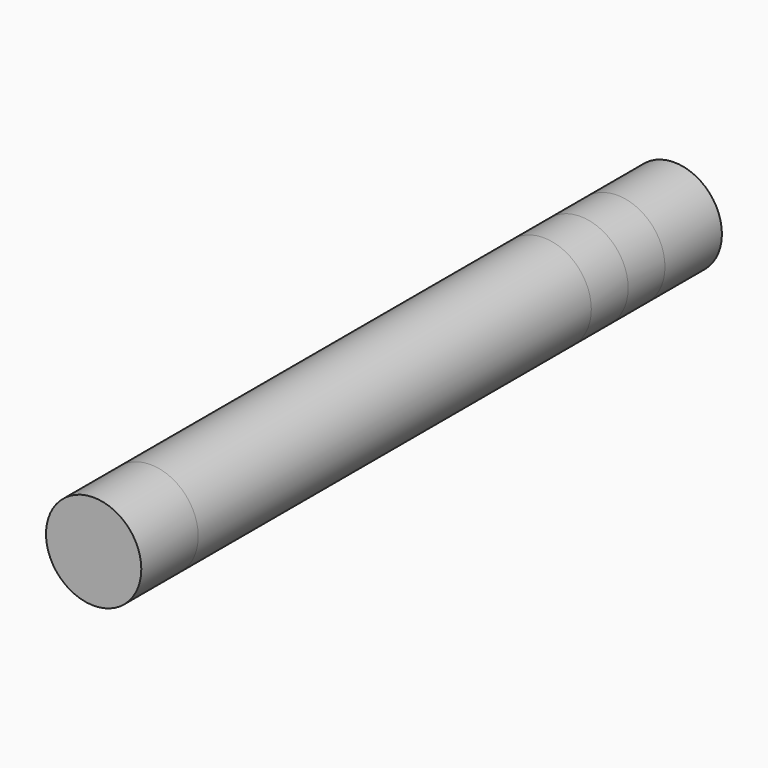
from build123d import *

# Parameters (mm, degrees)
F0_R          = 26.2972038965
F0_R_2        = 21.7596703079
F1_DEPTH      = 25.4
F2_DEPTH      = 25.4
F3_DEPTH      = 50.801
F3_DEPTH_BACK = 310.4061427


# Not quite as in the source:
# - an extrude ends at something that could not be found from the text; its depth is read off the source's solid
# - a feature of the source that left no trace in its solid (it failed there, or was rolled back) is left out
# - a pattern or mirror of a feature is missing from the dataset's text; its kind, count and spacing are read off the source's solid


with BuildPart() as f1:
    # F0 (on Front) → F1 (new body)
    with BuildSketch(Plane.XZ):
        with Locations((35.550635308, 42.1431325376)):
            Circle(F0_R)
        with Locations((35.550635308, 42.1431325376)):
            Circle(F0_R_2, mode=Mode.SUBTRACT)
        with Locations((35.550635308, 42.1431325376)):
            Circle(F0_R_2)
    extrude(amount=-F1_DEPTH)

    # F2 (add): a face of the model
    f2_faces = [f1.faces().sort_by_distance(p)[0] for p in [
        (35.550635308, 0, 42.1431325376),
    ]]
    extrude(f2_faces, amount=F2_DEPTH)

    # F3 (add, two sides): a face of the model
    f3_faces = [f1.faces().sort_by_distance(p)[0] for p in [
        (35.550635308, -25.4, 42.1431325376),
    ]]
    f3 = extrude(f3_faces, amount=-F3_DEPTH) + extrude(f3_faces, amount=F3_DEPTH_BACK)

    # F3_copies: F3 across plane
    add(f3.mirror(Plane.ZX.offset(-135.562021)))


solid = f1.part
